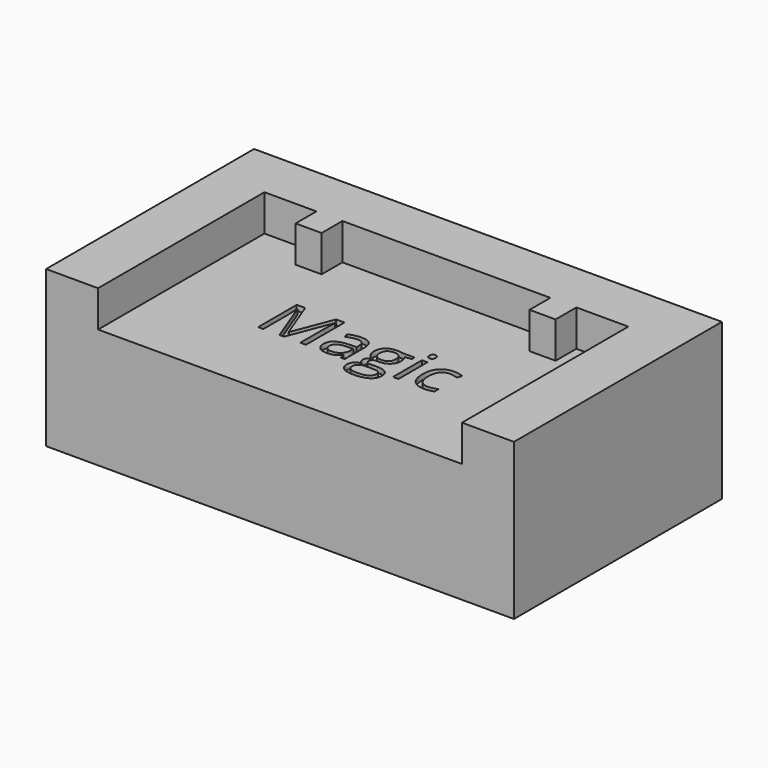
from build123d import *

# Parameters (mm, degrees)
F0_W         = 90
F0_H         = 50
F1_DEPTH     = 30
F2_W         = 70
F2_H         = 40
F3_DEPTH     = 7
F4_TEXT_SIZE = 13.0088645475
F5_DEPTH     = 1
F6_W         = 5
F6_H         = 7
F7_DEPTH     = 5


# Not quite as in the source:
# - Text() gives the source's letters only with a copy of the font that has no kerning and outlines rounded to 1/6400 em; it was checked with that copy


with BuildPart() as f1:
    # F0 (on Top) → F1 (new body)
    with BuildSketch(Plane.XY):
        with Locations((1.3525774702, -0.7706511484)):
            Rectangle(F0_W, F0_H)
    extrude(amount=F1_DEPTH)

    # F2 (on face) → F3 (cut)
    with BuildSketch(Plane.XY.offset(30)):
        with Locations((1.3525774702, -5.7706511484)):
            Rectangle(F2_W, F2_H)
    extrude(amount=-F3_DEPTH, mode=Mode.SUBTRACT)

    # F4 (on face) → F5 (cut)
    with BuildSketch(Plane.XY.offset(23)):
        with Locations((-16.6474225298, -10.1370336226)):
            Text('Magic', F4_TEXT_SIZE, font='Open Sans', text_align=(TextAlign.LEFT, TextAlign.BOTTOM))
    extrude(amount=-F5_DEPTH, mode=Mode.SUBTRACT)

    # F6 (on face) → F7 (join)
    with BuildSketch(Plane.XZ.offset(-14.2293488516)):
        with Locations((-21.1474225298, 26.5)):
            Rectangle(F6_W, F6_H)
        with Locations((23.8525774702, 26.5)):
            Rectangle(F6_W, F6_H)
    extrude(amount=F7_DEPTH)


solid = f1.part
